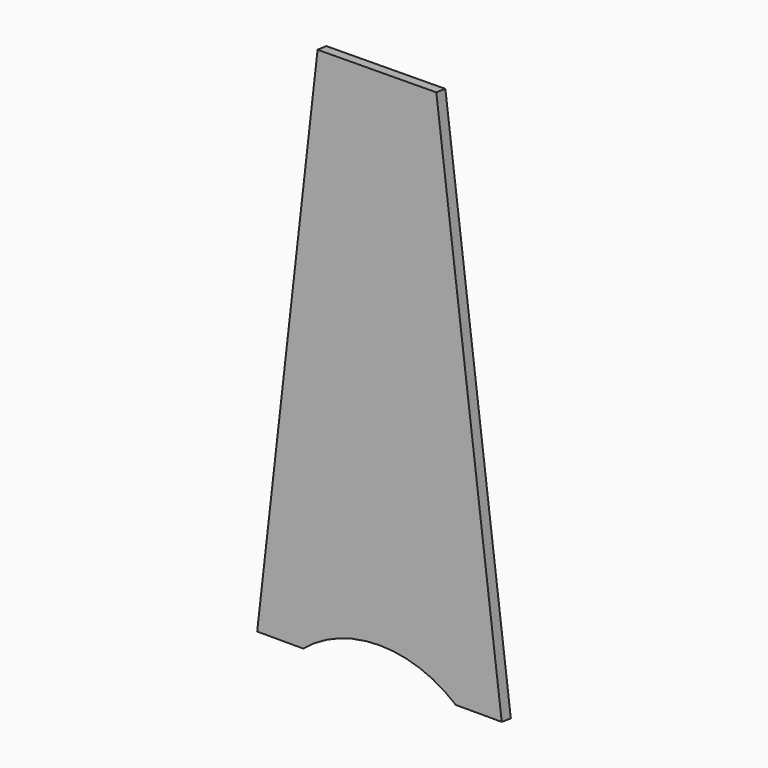
from build123d import *

# Parameters (mm, degrees)
F1_DEPTH = 19.05
F3_DEPTH = 19.05
F5_DEPTH = 419.1
F6_SIZE2 = 2.339036
F6_SIZE  = 19.04999


# Not quite as in the source:
# - a fillet or chamfer is up to 0.001 mm smaller than in the source, because OpenCascade refuses the exact size


with BuildPart() as f1:
    # F0 (on Front) → F1 (new body)
    with BuildSketch(Plane.XZ):
        Polygon((306.8257975104, 914.4), (103.6341967715, 912.5524640321), (0, 0), (419.1, 0), align=None)
    extrude(amount=F1_DEPTH)

    # F2 (on face) → F3 (cut)
    with BuildSketch(Plane.XZ.offset(19.05)):
        with BuildLine():
            Line((76.2, 0), (342.9, 0))
            ThreePointArc((342.9, 0), (209.55, 49.8767548608), (76.2, 0))
        make_face()
    extrude(amount=-F3_DEPTH, mode=Mode.SUBTRACT)

    # F4 (on Right) → F5 (cut)
    with BuildSketch(Plane.YZ):
        Polygon((-19.05, 2.3390458852), (-19.05, 0), (0, 0), align=None)
    extrude(amount=F5_DEPTH, mode=Mode.SUBTRACT)

    # F6 (size 19.05 and 2.3390458852 in the source; OpenCascade refuses exactly that, so slightly less here)
    f6_edges = [f1.edges().sort_by_distance(p)[0] for p in [
        (205.229997, 0, 913.476232),
    ]]
    f6_side = f1.faces().sort_by_distance((205.229997, -9.525, 913.476232))[0]
    chamfer(f6_edges, length=F6_SIZE, length2=F6_SIZE2, reference=f6_side)


solid = f1.part
